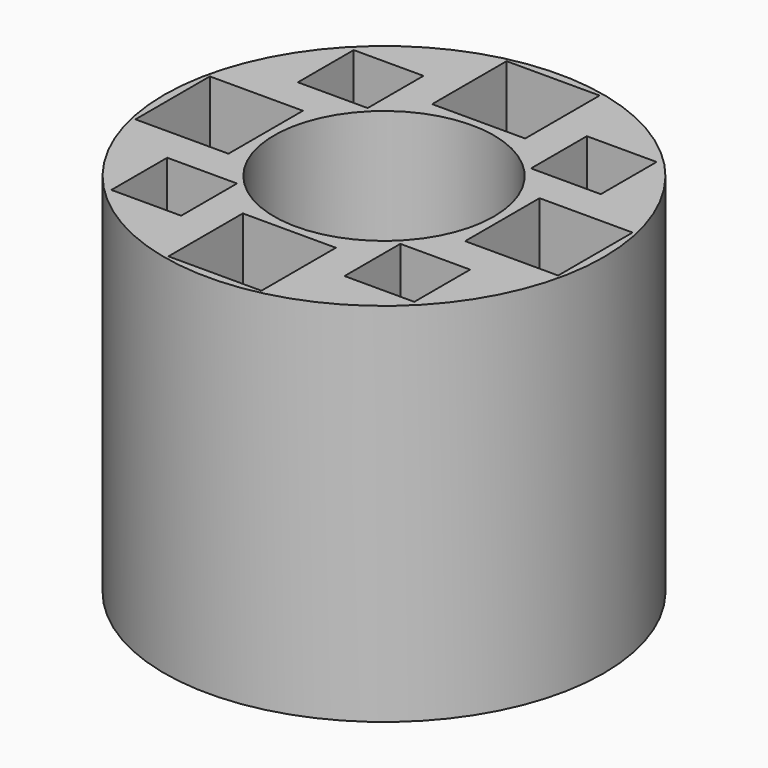
from build123d import *

# Parameters (mm, degrees)
F0_R            = 30
F0_R_2          = 15
F1_DEPTH        = 50
F2_W            = 12.7
F2_H            = 12.7
F3_DEPTH        = 50.001
F3_COPIES_COUNT = 4
F4_W            = 9.525
F4_H            = 9.525
F5_DEPTH        = 50.001
F5_COPIES_COUNT = 4


# Not quite as in the source:
# - a pattern or mirror of a feature is missing from the dataset's text; its kind, count and spacing are read off the source's solid


with BuildPart() as f1:
    # F0 (on Top) → F1 (new body)
    with BuildSketch(Plane.XY):
        Circle(F0_R)
        Circle(F0_R_2, mode=Mode.SUBTRACT)
    extrude(amount=F1_DEPTH)

    # F2 (on face) → F3 (cut, through all)
    with BuildSketch(Plane.XY.offset(50)):
        with Locations((0, 22.5)):
            Rectangle(F2_W, F2_H)
    f3 = extrude(amount=-F3_DEPTH, mode=Mode.SUBTRACT)

    # F3_copies: F3 ×4 about axis
    f3_copies_axis = Axis((0, 0, 0), (0, 0, 1))
    for i in range(1, F3_COPIES_COUNT):
        add(f3.rotate(f3_copies_axis, i * 360 / F3_COPIES_COUNT), mode=Mode.SUBTRACT)

    # F4 (on face) → F5 (cut, through all)
    with BuildSketch(Plane.XY.offset(50)):
        with Locations((-15.9099025767, 15.9099025767)):
            Rectangle(F4_W, F4_H)
    f5 = extrude(amount=-F5_DEPTH, mode=Mode.SUBTRACT)

    # F5_copies: F5 ×4 about axis
    f5_copies_axis = Axis((0, 0, 0), (0, 0, 1))
    for i in range(1, F5_COPIES_COUNT):
        add(f5.rotate(f5_copies_axis, i * 360 / F5_COPIES_COUNT), mode=Mode.SUBTRACT)


solid = f1.part
